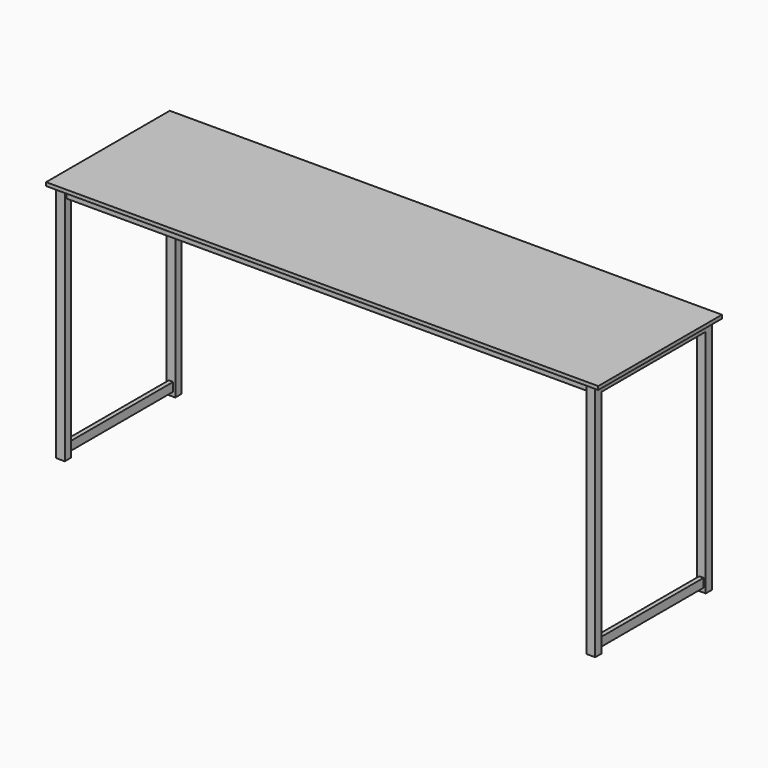
from build123d import *

# Parameters (mm, degrees)
F0_W     = 50.8
F0_H     = 45.1555665885
F0_W_2   = 40.64
F0_H_2   = 34.9955665885
F1_DEPTH = 1397
F2_W     = 25.4
F2_H     = 50.8
F2_W_2   = 15.24
F2_H_2   = 40.64
F2_W_3   = 50.8
F2_W_4   = 40.64
F3_DEPTH = 381
F4_W     = 19.7555665885
F4_H     = 50.8
F4_W_2   = 12.1355665885
F4_H_2   = 43.18
F5_DEPTH = 1524
F8_W     = 3225.8
F8_H     = 903.1111331769
F8_W_2   = 40.64
F8_H_2   = 34.9955665885
F8_W_3   = 3048
F8_H_3   = 787.4
F9_DEPTH = 20.32


with BuildPart() as f1:
    # F0 (on Top) → F1 (new body)
    with BuildSketch(Plane.XY):
        with Locations((-27.2679795849, -14.3071769268)):
            Rectangle(F0_W, F0_H)
        with Locations((-27.2679795849, -14.3071769268)):
            Rectangle(F0_W_2, F0_H_2, mode=Mode.SUBTRACT)
    extrude(amount=F1_DEPTH)

    # F2 (on face) → F3 (join)
    with BuildSketch(Plane(origin=(0, 8.2706063674, 0), x_dir=(-1, 0, 0), z_dir=(0, 1, 0))):
        with Locations((27.2679795849, 50.8)):
            Rectangle(F2_W, F2_H)
        with Locations((27.2679795849, 50.8)):
            Rectangle(F2_W_2, F2_H_2, mode=Mode.SUBTRACT)
        with Locations((27.2679795849, 1371.6)):
            Rectangle(F2_W_3, F2_H)
        with Locations((27.2679795849, 1371.6)):
            Rectangle(F2_W_4, F2_H_2, mode=Mode.SUBTRACT)
    extrude(amount=F3_DEPTH)

    # F4 (on face) → F5 (join)
    with BuildSketch(Plane.YZ.offset(-1.8679795849)):
        with Locations((-14.3071769268, 1371.6)):
            Rectangle(F4_W, F4_H)
        with Locations((-14.3071769268, 1371.6)):
            Rectangle(F4_W_2, F4_H_2, mode=Mode.SUBTRACT)
    extrude(amount=F5_DEPTH)

    # F6: F1 across face


with BuildPart() as f1_1:
    add(f1.part)
    add(f1.part.mirror(Plane(origin=(1522.1320204151, -14.3071769268, 1371.6), x_dir=(0, 1, 0), z_dir=(1, 0, 0))))

    # F7: F1 across face


with BuildPart() as f1_2:
    add(f1_1.part)
    add(f1_1.part.mirror(Plane(origin=(-27.2679795849, 389.2706063674, 1371.6), x_dir=(-1, 0, 0), z_dir=(0, 1, 0))))

    # F8 (on face) → F9 (join)
    with BuildSketch(Plane.XY.offset(1397)):
        with Locations((1522.1320204151, 389.2706063674)):
            Rectangle(F8_W, F8_H)
        Polygon((-52.6679795849, -36.8849602211), (-52.6679795849, 815.4261729559), (-1.8679795849, 815.4261729559), (-1.8679795849, 802.7261729559), (3046.1320204151, 802.7261729559), (3046.1320204151, 815.4261729559), (3096.9320204151, 815.4261729559), (3096.9320204151, -36.8849602211), (3046.1320204151, -36.8849602211), (3046.1320204151, -24.1849602211), (-1.8679795849, -24.1849602211), (-1.8679795849, -36.8849602211), align=None, mode=Mode.SUBTRACT)
        Polygon((-1.8679795849, 815.4261729559), (-52.6679795849, 815.4261729559), (-52.6679795849, -36.8849602211), (-1.8679795849, -36.8849602211), (-1.8679795849, -24.1849602211), (3046.1320204151, -24.1849602211), (3046.1320204151, -36.8849602211), (3096.9320204151, -36.8849602211), (3096.9320204151, 815.4261729559), (3046.1320204151, 815.4261729559), (3046.1320204151, 802.7261729559), (-1.8679795849, 802.7261729559), align=None)
        with Locations((-27.2679795849, -14.3071769268)):
            Rectangle(F8_W_2, F8_H_2, mode=Mode.SUBTRACT)
        with Locations((3071.5320204151, -14.3071769268)):
            Rectangle(F8_W_2, F8_H_2, mode=Mode.SUBTRACT)
        with Locations((1522.1320204151, 389.2706063674)):
            Rectangle(F8_W_3, F8_H_3, mode=Mode.SUBTRACT)
        with Locations((-27.2679795849, 792.8483896616)):
            Rectangle(F8_W_2, F8_H_2, mode=Mode.SUBTRACT)
        with Locations((3071.5320204151, 792.8483896616)):
            Rectangle(F8_W_2, F8_H_2, mode=Mode.SUBTRACT)
        with Locations((1522.1320204151, 389.2706063674)):
            Rectangle(F8_W_3, F8_H_3)
        with Locations((-27.2679795849, -14.3071769268)):
            Rectangle(F8_W_2, F8_H_2)
        with Locations((3071.5320204151, -14.3071769268)):
            Rectangle(F8_W_2, F8_H_2)
        with Locations((3071.5320204151, 792.8483896616)):
            Rectangle(F8_W_2, F8_H_2)
        with Locations((-27.2679795849, 792.8483896616)):
            Rectangle(F8_W_2, F8_H_2)
    extrude(amount=F9_DEPTH)


solid = f1_2.part
